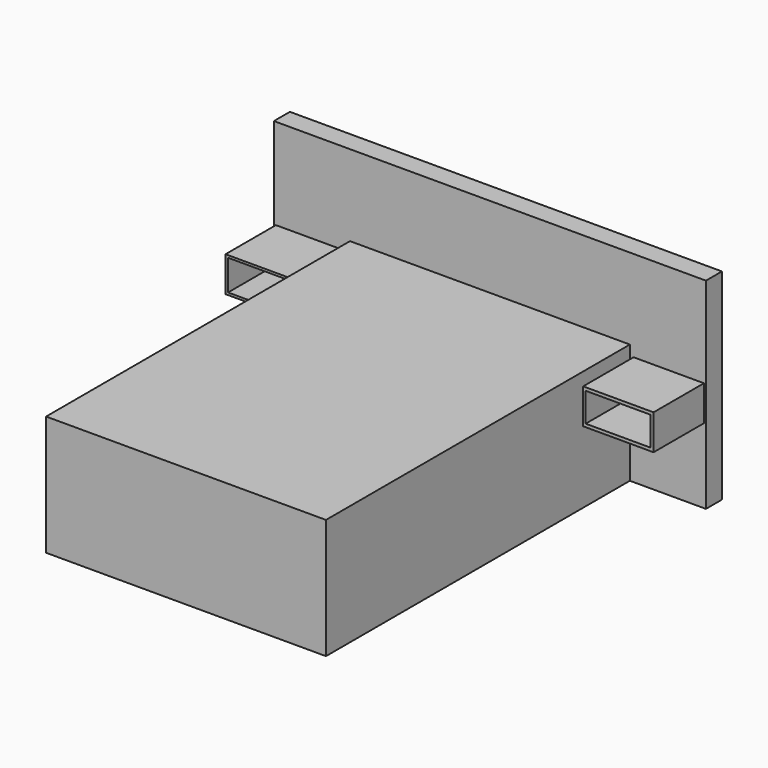
from build123d import *

# Parameters (mm, degrees)
F0_W      = 2161
F0_H      = 989
F1_DEPTH  = 16
F2_W      = 1400
F2_H      = 600
F3_DEPTH  = 1900
F4_W      = 352
F4_H      = 176
F5_DEPTH  = 315
F6_W      = 2161
F6_H      = 16
F7_DEPTH  = 100
F8_W      = 18
F8_H      = 971
F9_DEPTH  = 84
F11_W     = 326.9687574357
F11_H     = 152.7800559998
F12_DEPTH = 300
F13_W     = 323.2262134552
F13_H     = 144.838064909
F14_DEPTH = 300


# Not quite as in the source:
# - a feature names something its author has since deleted; it is built from what else it names


with BuildPart() as f1:
    # F0 (on Front) → F1 (new body)
    with BuildSketch(Plane.XZ):
        with Locations((1080.5, 494.5)):
            Rectangle(F0_W, F0_H)
    extrude(amount=F1_DEPTH)

    # F2 (on face) → F3 (join)
    with BuildSketch(Plane.XZ.offset(16)):
        with Locations((1080.5, 300)):
            Rectangle(F2_W, F2_H)
    extrude(amount=F3_DEPTH)

    # F4 (on face) → F5 (join)
    with BuildSketch(Plane.XZ.offset(16)):
        with Locations((186, 462)):
            Rectangle(F4_W, F4_H)
        with Locations((1975, 462)):
            Rectangle(F4_W, F4_H)
    extrude(amount=F5_DEPTH)

    # F6 (on face) → F7 (join)
    with BuildSketch(Plane.XZ.offset(16)):
        with Locations((1080.5, 997)):
            Rectangle(F6_W, F6_H)
    extrude(amount=-F7_DEPTH)

    # F8 (on face) → F9 (join)
    with BuildSketch(Plane(origin=(0, 0, 0), x_dir=(-1, 0, 0), z_dir=(0, 1, 0))):
        Polygon((-2161, 18), (-2161, 0), (0, 0), (0, 18), (-18, 18), (-1091.649181366, 18), (-1109.649181366, 18), (-1478.5152740479, 18), (-1496.5152740479, 18), (-2143, 18), align=None)
        with Locations((-2152, 503.5)):
            Rectangle(F8_W, F8_H)
        with Locations((-9, 503.5)):
            Rectangle(F8_W, F8_H)
        with Locations((-1100.649181366, 503.5)):
            Rectangle(F8_W, F8_H)
    extrude(amount=F9_DEPTH)

    # F11 (on face) → F12 (cut)
    with BuildSketch(Plane.XZ.offset(331)):
        with Locations((186.2288573757, 462.0463848114)):
            Rectangle(F11_W, F11_H)
    extrude(amount=-F12_DEPTH, mode=Mode.SUBTRACT)

    # F13 (on face) → F14 (cut)
    with BuildSketch(Plane.XZ.offset(331)):
        with Locations((1973.0969667435, 461.9913846254)):
            Rectangle(F13_W, F13_H)
    extrude(amount=-F14_DEPTH, mode=Mode.SUBTRACT)


solid = f1.part
